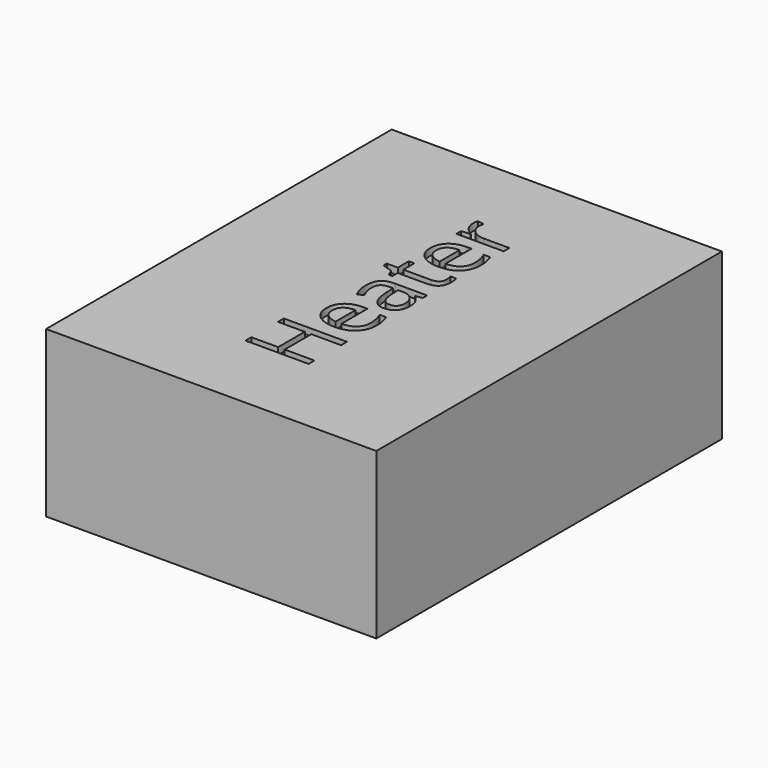
from build123d import *

# Parameters (mm, degrees)
F0_W         = 304.8
F0_H         = 398.78
F1_DEPTH     = 152.4
F2_TEXT_SIZE = 81.6522678654
F3_DEPTH     = 6.35


# Not quite as in the source:
# - Text() gives the source's letters only with a copy of the font that has no kerning and outlines rounded to 1/6400 em; it was checked with that copy


with BuildPart() as f1:
    # F0 (on Top) → F1 (new body)
    with BuildSketch(Plane.XY):
        with Locations((152.4, 199.39)):
            Rectangle(F0_W, F0_H)
    extrude(amount=F1_DEPTH)

    # F2 (on face) → F3 (cut)
    with BuildSketch(Plane.XY.offset(152.4)):
        with Locations(Location((181.7948164315, 67.604515482), (0, 0, 90))):
            Text('Heater', F2_TEXT_SIZE, font='Open Sans', text_align=(TextAlign.LEFT, TextAlign.BOTTOM))
    extrude(amount=-F3_DEPTH, mode=Mode.SUBTRACT)


solid = f1.part
